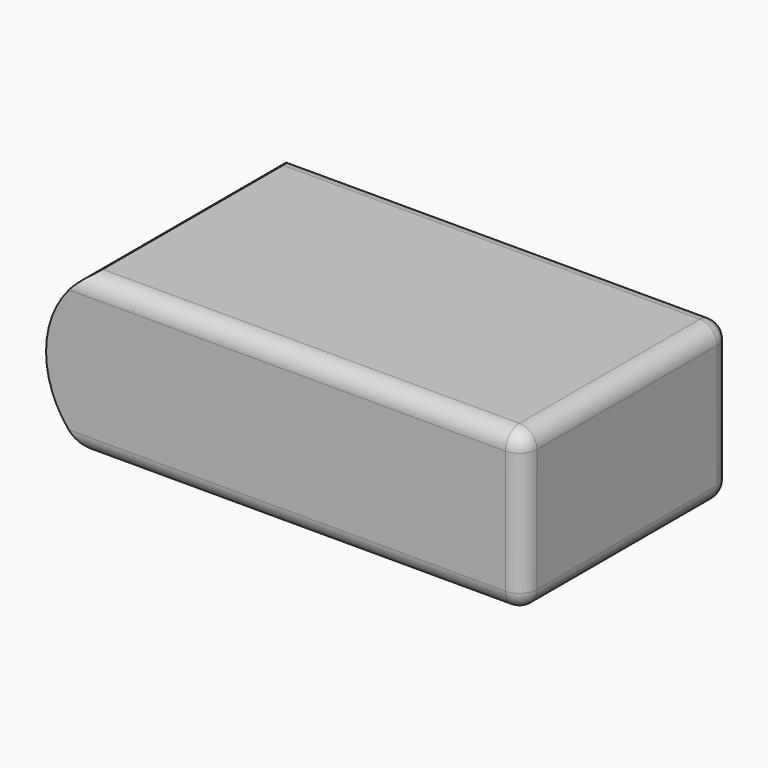
from build123d import *

# Parameters (mm, degrees)
F1_DEPTH = 14.925
F2_R     = 2


with BuildPart() as f1:
    # F0 (on Front) → F1 (new body, symmetric)
    with BuildSketch(Plane.XZ):
        with BuildLine():
            Line((-22.5191842765, -9.075), (27.365, -9.075))
            Line((27.365, -9.075), (27.365, 9.075))
            Line((27.365, 9.075), (-22.4661100656, 9.075))
            ThreePointArc((-22.4661100656, 9.075), (-26.0623595245, 5.1465764849), (-27.3650142087, -0.0175896876))
            ThreePointArc((-27.3650142087, -0.0175896876), (-26.0774195294, -5.1537056642), (-22.5191842765, -9.075))
        make_face()
    extrude(amount=F1_DEPTH, both=True)

    # F2
    f2_edges = [f1.edges().sort_by_distance(p)[0] for p in [
        (2.449445, -14.925, 9.075),
        (2.449445, 14.925, 9.075),
        (27.365, 7.4625, 9.075),
        (27.365, -7.4625, 9.075),
        (-22.519184, 7.4625, -9.075),
        (2.422908, 14.925, -9.075),
        (27.365, 7.4625, -9.075),
        (27.365, -7.4625, -9.075),
        (2.422908, -14.925, -9.075),
        (-22.519184, -7.4625, -9.075),
        (27.365, -14.925, 0),
        (27.365, 14.925, 0),
    ]]
    fillet(f2_edges, radius=F2_R)


solid = f1.part
